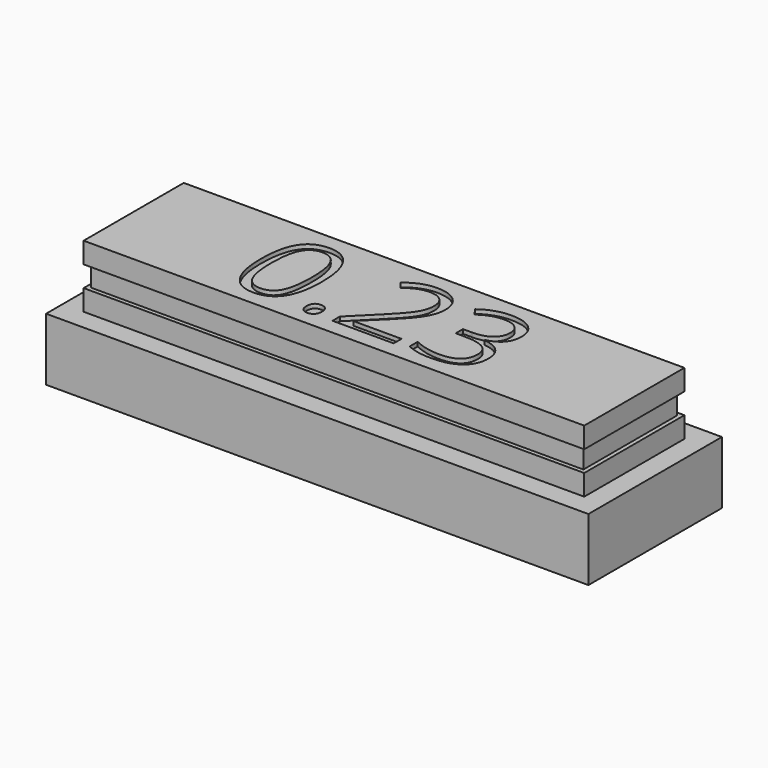
from build123d import *

# Parameters (mm, degrees)
F0_W         = 26
F0_H         = 8
F0_W_2       = 20
F0_H_2       = 2
F1_DEPTH     = 3
F2_W         = 24
F2_H         = 6
F3_DEPTH     = 3
F5_W         = 24
F5_H         = 6
F5_W_2       = 23.6
F5_H_2       = 5.6
F6_DEPTH     = 0.5
F7_W         = 19.54
F7_H         = 1.54
F8_DEPTH     = 3
F9_TEXT_SIZE = 6.25
F10_DEPTH    = 0.2


# Not quite as in the source:
# - Text() gives the source's letters only with a copy of the font that has no kerning and outlines rounded to 1/6400 em; it was checked with that copy


with BuildPart() as f1:
    # F0 (on Top) → F1 (new body)
    with BuildSketch(Plane.XY):
        Rectangle(F0_W, F0_H)
        Rectangle(F0_W_2, F0_H_2, mode=Mode.SUBTRACT)
    extrude(amount=F1_DEPTH)


with BuildPart() as f3:
    # F2 (on face) → F3 (new body)
    with BuildSketch(Plane.XY.offset(3)):
        Rectangle(F2_W, F2_H)
    extrude(amount=F3_DEPTH)

    # F5 (on mid) → F6 (cut, symmetric)
    with BuildSketch(Plane.XY.offset(4.5)):
        Rectangle(F5_W, F5_H)
        Rectangle(F5_W_2, F5_H_2, mode=Mode.SUBTRACT)
    extrude(amount=F6_DEPTH, both=True, mode=Mode.SUBTRACT)

    # F7 (on face) → F8 (join, through all)
    with BuildSketch(Plane(origin=(0, 0, 3), x_dir=(1, 0, 0), z_dir=(0, 0, -1))):
        Rectangle(F7_W, F7_H)
    extrude(amount=F8_DEPTH)

    # F9 (on face) → F10 (cut)
    with BuildSketch(Plane.XY.offset(6)):
        with Locations((-6.2109375, -2.25)):
            Text('0.23', F9_TEXT_SIZE, font='Open Sans', text_align=(TextAlign.LEFT, TextAlign.BOTTOM))
    extrude(amount=-F10_DEPTH, mode=Mode.SUBTRACT)


solid = Compound([f1.part, f3.part])
